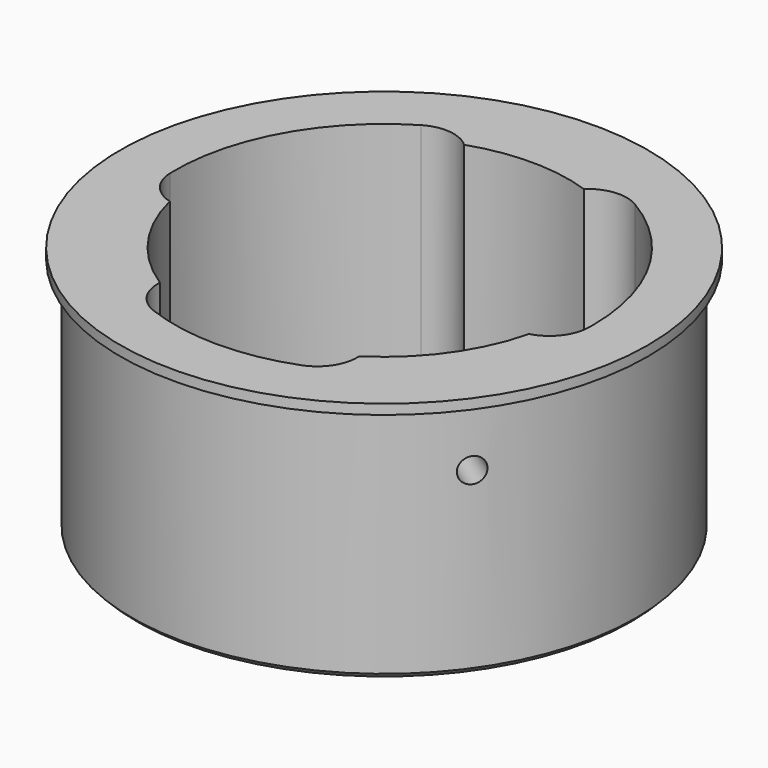
from build123d import *

# Parameters (mm, degrees)
F0_R           = 26.5
F0_R_2         = 25.3
F1_DEPTH       = 1
F2_DEPTH       = 25
F3_DEPTH       = 22
F4_T1_DEPTH    = 22
F9_D           = 2.5
F9_DEPTH       = 25
F9_START       = 1.2308984
F9_TIP         = 0.7510757738
F9_ON_F7_D     = 2.5
F9_ON_F7_DEPTH = 25
F9_ON_F7_START = 1.2308984
F9_ON_F7_TIP   = 0.7510757738
F10_SIZE       = 0.5


# Not quite as in the source:
# - a fillet or chamfer that OpenCascade refuses, or shapes differently, is made with other operations: its cross-section is extruded or revolved along the edge and cut away or added


with BuildPart() as f1:
    # F0 (on Top) → F1 (new body)
    with BuildSketch(Plane.XY):
        Circle(F0_R)
        Circle(F0_R_2, mode=Mode.SUBTRACT)
        Circle(F0_R_2)
        with BuildLine():
            ThreePointArc((-6.7924528302, 19.8711495528), (0, 21), (6.7924528302, 19.8711495528))
            ThreePointArc((6.7924528302, 19.8711495528), (17.0827619171, 12.2138955818), (21, 0))
            ThreePointArc((21, 0), (20.8522276614, -2.4868859159), (20.4109903277, -4.9387725035))
            ThreePointArc((20.4109903277, -4.9387725035), (17.0984542242, -12.1919179436), (11.320754717, -17.6872980593))
            ThreePointArc((11.320754717, -17.6872980593), (0, -21), (-11.320754717, -17.6872980593))
            ThreePointArc((-11.320754717, -17.6872980593), (-17.0984542242, -12.1919179436), (-20.4109903277, -4.9387725035))
            ThreePointArc((-20.4109903277, -4.9387725035), (-18.4089621658, 10.1049548232), (-6.7924528302, 19.8711495528))
        make_face(mode=Mode.SUBTRACT)
    extrude(amount=-F1_DEPTH)

    # F0 (on Top) → F2 (join)
    with BuildSketch(Plane.XY):
        Circle(F0_R_2)
        with BuildLine():
            ThreePointArc((-6.7924528302, 19.8711495528), (0, 21), (6.7924528302, 19.8711495528))
            ThreePointArc((6.7924528302, 19.8711495528), (17.0827619171, 12.2138955818), (21, 0))
            ThreePointArc((21, 0), (20.8522276614, -2.4868859159), (20.4109903277, -4.9387725035))
            ThreePointArc((20.4109903277, -4.9387725035), (17.0984542242, -12.1919179436), (11.320754717, -17.6872980593))
            ThreePointArc((11.320754717, -17.6872980593), (0, -21), (-11.320754717, -17.6872980593))
            ThreePointArc((-11.320754717, -17.6872980593), (-17.0984542242, -12.1919179436), (-20.4109903277, -4.9387725035))
            ThreePointArc((-20.4109903277, -4.9387725035), (-18.4089621658, 10.1049548232), (-6.7924528302, 19.8711495528))
        make_face(mode=Mode.SUBTRACT)
        with BuildLine():
            Line((20.4109903277, -4.9387725035), (18.0297081228, -4.3625823781))
            ThreePointArc((18.0297081228, -4.3625823781), (15.1036345647, -10.7695275168), (10, -15.6237799524))
            Line((10, -15.6237799524), (11.320754717, -17.6872980593))
            ThreePointArc((11.320754717, -17.6872980593), (17.0984542242, -12.1919179436), (20.4109903277, -4.9387725035))
        make_face()
        with BuildLine():
            ThreePointArc((6, 17.5528487716), (15.0897730268, 10.7889410973), (18.55, 0))
            ThreePointArc((18.55, 0), (18.4194677675, -2.1967492257), (18.0297081228, -4.3625823781))
            Line((18.0297081228, -4.3625823781), (20.4109903277, -4.9387725035))
            ThreePointArc((20.4109903277, -4.9387725035), (20.8522276614, -2.4868859159), (21, 0))
            ThreePointArc((21, 0), (17.0827619171, 12.2138955818), (6.7924528302, 19.8711495528))
            Line((6.7924528302, 19.8711495528), (6, 17.5528487716))
        make_face()
        with BuildLine():
            ThreePointArc((-6, 17.5528487716), (0, 18.55), (6, 17.5528487716))
            Line((6, 17.5528487716), (6.7924528302, 19.8711495528))
            ThreePointArc((6.7924528302, 19.8711495528), (0, 21), (-6.7924528302, 19.8711495528))
            Line((-6.7924528302, 19.8711495528), (-6, 17.5528487716))
        make_face()
        with BuildLine():
            ThreePointArc((-18.0297081228, -4.3625823781), (-16.2612499131, 8.9260434271), (-6, 17.5528487716))
            Line((-6, 17.5528487716), (-6.7924528302, 19.8711495528))
            ThreePointArc((-6.7924528302, 19.8711495528), (-18.4089621658, 10.1049548232), (-20.4109903277, -4.9387725035))
            Line((-20.4109903277, -4.9387725035), (-18.0297081228, -4.3625823781))
        make_face()
        with BuildLine():
            ThreePointArc((-10, -15.6237799524), (-15.1036345647, -10.7695275168), (-18.0297081228, -4.3625823781))
            Line((-18.0297081228, -4.3625823781), (-20.4109903277, -4.9387725035))
            ThreePointArc((-20.4109903277, -4.9387725035), (-17.0984542242, -12.1919179436), (-11.320754717, -17.6872980593))
            Line((-11.320754717, -17.6872980593), (-10, -15.6237799524))
        make_face()
        with BuildLine():
            Line((11.320754717, -17.6872980593), (10, -15.6237799524))
            ThreePointArc((10, -15.6237799524), (0, -18.55), (-10, -15.6237799524))
            Line((-10, -15.6237799524), (-11.320754717, -17.6872980593))
            ThreePointArc((-11.320754717, -17.6872980593), (0, -21), (11.320754717, -17.6872980593))
        make_face()
    extrude(amount=-F2_DEPTH)

    # F0 (on Top) → F3 (cut)
    with BuildSketch(Plane.XY):
        with BuildLine():
            ThreePointArc((6, 17.5528487716), (15.0897730268, 10.7889410973), (18.55, 0))
            ThreePointArc((18.55, 0), (18.4194677675, -2.1967492257), (18.0297081228, -4.3625823781))
            Line((18.0297081228, -4.3625823781), (20.4109903277, -4.9387725035))
            ThreePointArc((20.4109903277, -4.9387725035), (20.8522276614, -2.4868859159), (21, 0))
            ThreePointArc((21, 0), (17.0827619171, 12.2138955818), (6.7924528302, 19.8711495528))
            Line((6.7924528302, 19.8711495528), (6, 17.5528487716))
        make_face()
        with BuildLine():
            Line((11.320754717, -17.6872980593), (10, -15.6237799524))
            ThreePointArc((10, -15.6237799524), (0, -18.55), (-10, -15.6237799524))
            Line((-10, -15.6237799524), (-11.320754717, -17.6872980593))
            ThreePointArc((-11.320754717, -17.6872980593), (0, -21), (11.320754717, -17.6872980593))
        make_face()
        with BuildLine():
            ThreePointArc((-18.0297081228, -4.3625823781), (-16.2612499131, 8.9260434271), (-6, 17.5528487716))
            Line((-6, 17.5528487716), (-6.7924528302, 19.8711495528))
            ThreePointArc((-6.7924528302, 19.8711495528), (-18.4089621658, 10.1049548232), (-20.4109903277, -4.9387725035))
            Line((-20.4109903277, -4.9387725035), (-18.0297081228, -4.3625823781))
        make_face()
    extrude(amount=-F3_DEPTH, mode=Mode.SUBTRACT)

    # F4: fillet of radius 4 on 6 edges, made by hand

    # F4_s2 → F4_t1 (join)
    with BuildSketch(Plane.XY.offset(-22)):
        with BuildLine():
            ThreePointArc((10.7499670552, 18.0399059951), (8.2943373762, 18.582869286), (6, 17.5528487716))
            Line((6, 17.5528487716), (5.9459529143, 17.6118310786))
            ThreePointArc((5.9459529143, 17.6118310786), (6.3205267978, 18.737875173), (6.7167532128, 19.8970255636))
            Line((6.7167532128, 19.8970255636), (6.818328841, 19.9468491701))
            ThreePointArc((6.818328841, 19.9468491701), (8.852466778, 19.1311325317), (10.7909193107, 18.1086294465))
            Line((10.7909193107, 18.1086294465), (10.7499670552, 18.0399059951))
        make_face()
        with BuildLine():
            ThreePointArc((-6, 17.5528487716), (-8.2943373762, 18.582869286), (-10.7499670552, 18.0399059951))
            Line((-10.7499670552, 18.0399059951), (-10.7909193107, 18.1086294465))
            ThreePointArc((-10.7909193107, 18.1086294465), (-8.852466778, 19.1311325317), (-6.818328841, 19.9468491701))
            Line((-6.818328841, 19.9468491701), (-6.7167532128, 19.8970255636))
            ThreePointArc((-6.7167532128, 19.8970255636), (-6.3205267978, 18.737875173), (-5.9459529143, 17.6118310786))
            Line((-5.9459529143, 17.6118310786), (-6, 17.5528487716))
        make_face()
        with BuildLine():
            ThreePointArc((18.0297081228, -4.3625823781), (20.1305359874, -2.9800309182), (20.9909384883, -0.6168479392))
            Line((20.9909384883, -0.6168479392), (21.0709039683, -0.6191978361))
            ThreePointArc((21.0709039683, -0.6191978361), (20.8927389597, -2.8035439649), (20.4887464814, -4.957586875))
            Line((20.4887464814, -4.957586875), (20.3921759563, -5.0165286572))
            ThreePointArc((20.3921759563, -5.0165286572), (19.2015348538, -4.7284335945), (18.0504489955, -4.4398469638))
            Line((18.0504489955, -4.4398469638), (18.0297081228, -4.3625823781))
        make_face()
        with BuildLine():
            ThreePointArc((7.423758192, -19.6440274462), (9.3775452078, -18.0604736729), (10, -15.6237799524))
            Line((10, -15.6237799524), (10.0798058197, -15.6182093928))
            ThreePointArc((10.0798058197, -15.6182093928), (10.7277575416, -16.6124123212), (11.3881349001, -17.6441713746))
            Line((11.3881349001, -17.6441713746), (11.3638814016, -17.7546782424))
            ThreePointArc((11.3638814016, -17.7546782424), (9.4590814084, -18.8385821895), (7.4520391756, -19.7188618365))
            Line((7.4520391756, -19.7188618365), (7.423758192, -19.6440274462))
        make_face()
        with BuildLine():
            ThreePointArc((-10, -15.6237799524), (-9.3775452078, -18.0604736729), (-7.423758192, -19.6440274462))
            Line((-7.423758192, -19.6440274462), (-7.4520391756, -19.7188618365))
            ThreePointArc((-7.4520391756, -19.7188618365), (-9.4590814084, -18.8385821895), (-11.3638814016, -17.7546782424))
            Line((-11.3638814016, -17.7546782424), (-11.3881349001, -17.6441713746))
            ThreePointArc((-11.3881349001, -17.6441713746), (-10.7277575416, -16.6124123212), (-10.0798058197, -15.6182093928))
            Line((-10.0798058197, -15.6182093928), (-10, -15.6237799524))
        make_face()
        with BuildLine():
            ThreePointArc((-20.9909384883, -0.6168479392), (-20.1305359874, -2.9800309182), (-18.0297081228, -4.3625823781))
            Line((-18.0297081228, -4.3625823781), (-18.0504489955, -4.4398469638))
            ThreePointArc((-18.0504489955, -4.4398469638), (-19.2015348538, -4.7284335945), (-20.3921759563, -5.0165286572))
            Line((-20.3921759563, -5.0165286572), (-20.4887464814, -4.957586875))
            ThreePointArc((-20.4887464814, -4.957586875), (-20.8927389597, -2.8035439649), (-21.0709039683, -0.6191978361))
            Line((-21.0709039683, -0.6191978361), (-20.9909384883, -0.6168479392))
        make_face()
    extrude(amount=F4_T1_DEPTH)

    # F9
    # its depths count from where the whole tool has entered the part; down to there all is cleared
    with Locations(Plane(origin=(-21.5766208067, -15.3850393098, 0), x_dir=(0.5805675211, -0.8142121059, 0), z_dir=(-0.8142121059, -0.5805675211, 0)).offset(-F9_START)):
        with Locations((0, -7)):
            Hole(F9_D / 2, depth=F9_DEPTH)
            with Locations((0, 0, -(F9_DEPTH + F9_TIP / 2))):  # 118° drill point
                Cone(0, F9_D / 2, F9_TIP, mode=Mode.SUBTRACT)

    # F9 on F7
    # its depths count from where the whole tool has entered the part; down to there all is cleared
    with Locations(Plane(origin=(21.5766208067, -15.3850393098, 0), x_dir=(0.5805675211, 0.8142121059, 0), z_dir=(0.8142121059, -0.5805675211, 0)).offset(-F9_ON_F7_START)):
        with Locations((0, -7)):
            Hole(F9_ON_F7_D / 2, depth=F9_ON_F7_DEPTH)
            with Locations((0, 0, -(F9_ON_F7_DEPTH + F9_ON_F7_TIP / 2))):  # 118° drill point
                Cone(0, F9_ON_F7_D / 2, F9_ON_F7_TIP, mode=Mode.SUBTRACT)

    # F10
    f10_edges = [f1.edges().sort_by_distance(p)[0] for p in [
        (-10, 15.62378, -25),
        (-25.3, 0, -25),
    ]]
    chamfer(f10_edges, length=F10_SIZE)


solid = f1.part
